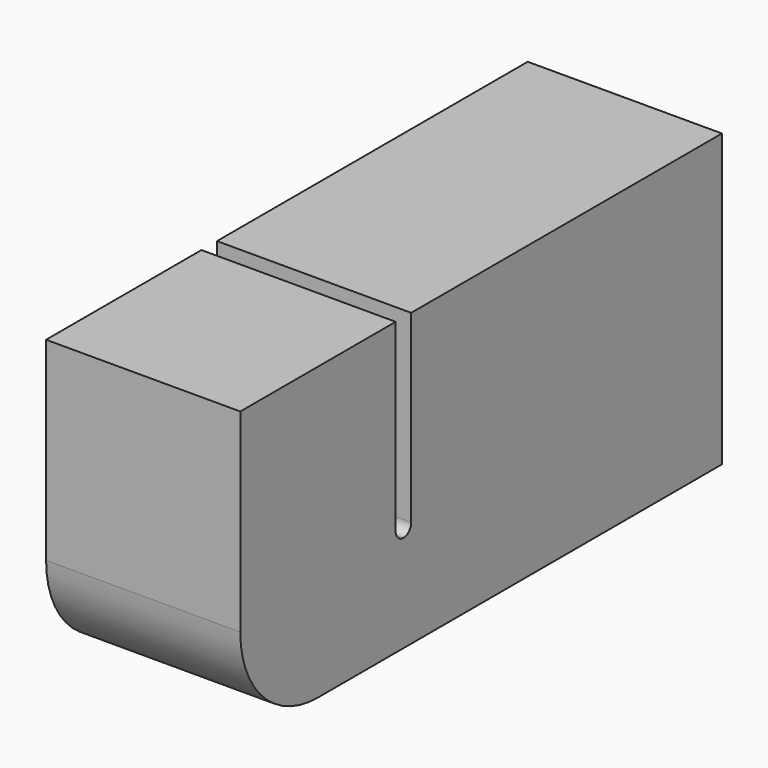
from build123d import *

# Parameters (mm, degrees)
F0_W     = 1
F0_H     = 5
F1_DEPTH = 10
F2_R     = 0.49999


# Not quite as in the source:
# - a fillet or chamfer is up to 0.001 mm smaller than in the source, because OpenCascade refuses the exact size


with BuildPart() as f1:
    # F0 (on Right) → F1 (new body)
    with BuildSketch(Plane.YZ):
        Polygon((20, -5), (20, 10), (0, 10), (0, 0), (0, -5), align=None)
        with Locations((-0.5, -2.5)):
            Rectangle(F0_W, F0_H)
        with BuildLine():
            Line((-1, -5), (-1, 0))
            Line((-1, 0), (-1, 10))
            Line((-1, 10), (-11, 10))
            Line((-11, 10), (-11, 0))
            ThreePointArc((-11, 0), (-9.5355339059, -3.5355339059), (-6, -5))
            Line((-6, -5), (-1, -5))
        make_face()
    extrude(amount=F1_DEPTH)

    # F2 (radius 0.5 in the source; OpenCascade refuses exactly that, so slightly less here)
    f2_edges = [f1.edges().sort_by_distance(p)[0] for p in [
        (5, 0, 0),
        (5, -1, 0),
    ]]
    fillet(f2_edges, radius=F2_R)


solid = f1.part
